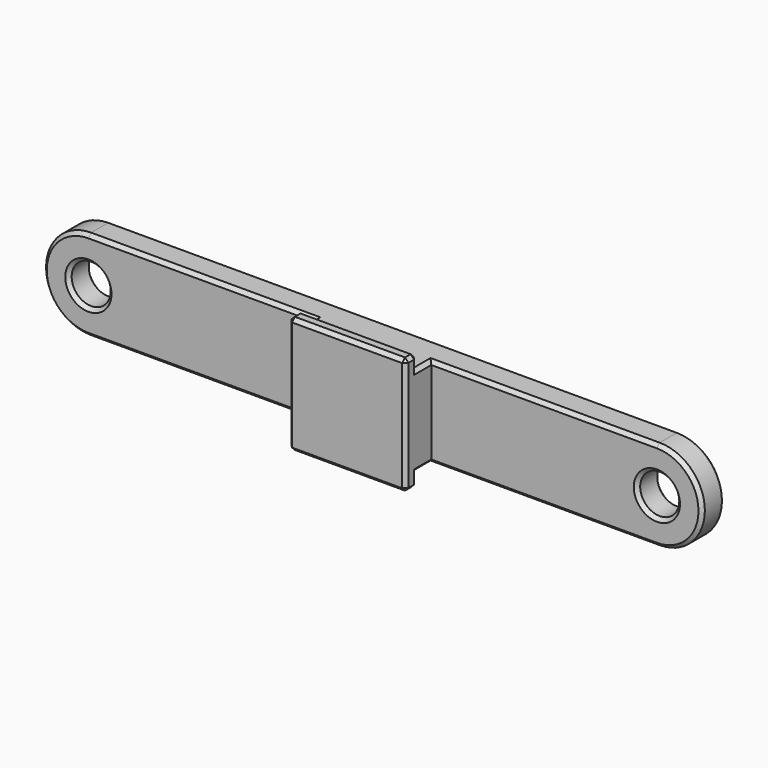
from build123d import *

# Parameters (mm, degrees)
F0_R     = 2.75
F1_DEPTH = 4
F2_W     = 16.5
F2_H     = 16.5
F3_DEPTH = 4.5
F4_W     = 26.5
F4_H     = 22.7
F4_W_2   = 16.5
F4_H_2   = 12.7
F5_DEPTH = 2.5
F7_SIZE  = 0.5


with BuildPart() as f1:
    # F0 (on Front) → F1 (new body)
    with BuildSketch(Plane.XZ):
        with BuildLine():
            ThreePointArc((40, -6.35), (46.35, 0), (40, 6.35))
            Line((40, 6.35), (-40, 6.35))
            ThreePointArc((-40, 6.35), (-46.35, 0), (-40, -6.35))
            Line((-40, -6.35), (40, -6.35))
        make_face()
        with Locations((-40, 0)):
            Circle(F0_R, mode=Mode.SUBTRACT)
        with Locations((40, 0)):
            Circle(F0_R, mode=Mode.SUBTRACT)
    extrude(amount=-F1_DEPTH)

    # F2 (on Front) → F3 (join)
    with BuildSketch(Plane.XZ):
        Rectangle(F2_W, F2_H)
    extrude(amount=F3_DEPTH)

    # F4 (on face) → F5 (cut)
    with BuildSketch(Plane.XZ):
        Rectangle(F4_W, F4_H)
        Rectangle(F4_W_2, F4_H_2, mode=Mode.SUBTRACT)
    extrude(amount=F5_DEPTH, mode=Mode.SUBTRACT)

    # F7
    f7_edges = [f1.edges().sort_by_distance(p)[0] for p in [
        (8.25, -4.5, 0),
        (0, -4.5, 8.25),
        (-8.25, -4.5, 0),
        (0, -4.5, -8.25),
        (8.25, -3.5, 8.25),
        (-8.25, -3.5, 8.25),
        (-8.25, -3.5, -8.25),
        (8.25, -3.5, -8.25),
        (46.35, 4, 0),
        (0, 4, 6.35),
        (-46.35, 4, 0),
        (0, 4, -6.35),
        (-42.75, 4, 0),
        (37.25, 4, 0),
        (0, -2.5, 8.25),
        (8.25, -2.5, -7.3),
        (8.25, -2.5, 7.3),
        (-8.25, -2.5, 7.3),
        (-8.25, -2.5, -7.3),
        (0, -2.5, -8.25),
        (24.125, 0, 6.35),
        (37.25, 0, 0),
        (8.25, -1.25, 6.35),
        (8.25, -1.25, -6.35),
        (-8.25, -1.25, 6.35),
        (-8.25, -1.25, -6.35),
        (-24.125, 0, -6.35),
        (-42.75, 0, 0),
        (46.35, 0, 0),
        (-46.35, 0, 0),
        (-24.125, 0, 6.35),
        (24.125, 0, -6.35),
    ]]
    chamfer(f7_edges, length=F7_SIZE)


solid = f1.part
